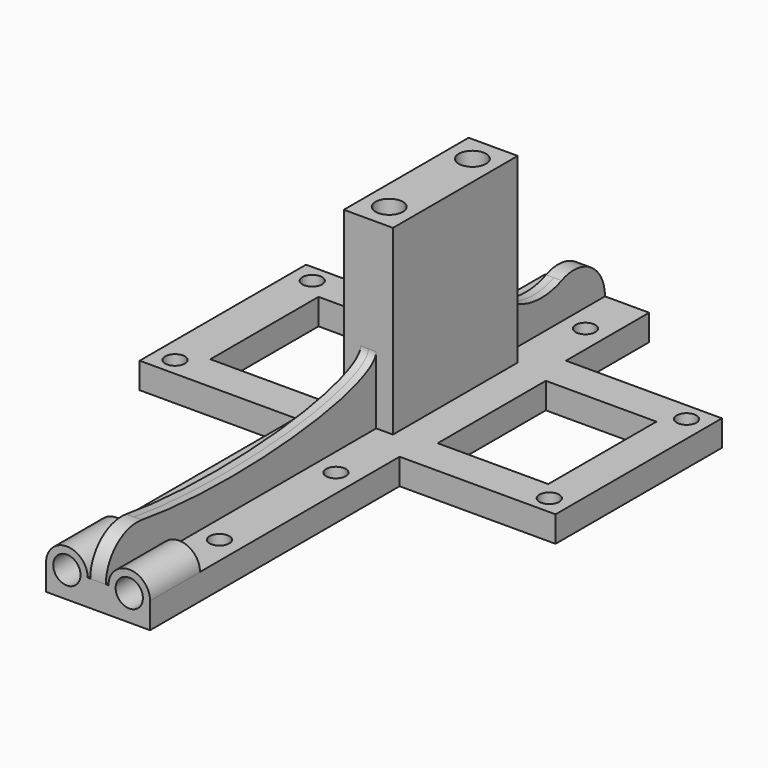
from build123d import *

# Parameters (mm, degrees)
F0_W      = 12
F0_H      = 38.1
F1_DEPTH  = 50.8
F2_R      = 3.33175
F3_DEPTH  = 25.4
F4_W      = 25.4
F4_H      = 76.2
F4_W_2    = 38.1
F4_H_2    = 50.8
F4_W_3    = 12
F4_H_3    = 38.1
F4_H_4    = 25.4
F5_DEPTH  = 6.35
F7_DEPTH  = 1.905
F8_R      = 3.33175
F9_DEPTH  = 12.7
F10_R     = 5.08
F11_DEPTH = 15.24
F13_DEPTH = 2.54
F14_W     = 27.02
F14_H     = 33.02
F15_DEPTH = 6.351
F16_R     = 2.413
F17_DEPTH = 6.351


# Not quite as in the source:
# - a pattern or mirror of a feature is missing from the dataset's text; its kind, count and spacing are read off the source's solid


with BuildPart() as f1:
    # F0 (on Top) → F1 (new body)
    with BuildSketch(Plane.XY):
        Rectangle(F0_W, F0_H)
    extrude(amount=F1_DEPTH)

    # F2 (on face) → F3 (cut)
    with BuildSketch(Plane.XY.offset(50.8)):
        with Locations((0, 12.7)):
            Circle(F2_R)
        with Locations((0, -12.7)):
            Circle(F2_R)
    extrude(amount=-F3_DEPTH, mode=Mode.SUBTRACT)

    # F4 (on face) → F5 (join)
    with BuildSketch(Plane(origin=(0, 0, 0), x_dir=(1, 0, 0), z_dir=(0, 0, -1))):
        with Locations((0, 63.5)):
            Rectangle(F4_W, F4_H)
        with Locations((31.75, 0)):
            Rectangle(F4_W_2, F4_H_2)
        Rectangle(F4_W, F4_H_2)
        Rectangle(F4_W_3, F4_H_3, mode=Mode.SUBTRACT)
        with Locations((-31.75, 0)):
            Rectangle(F4_W_2, F4_H_2)
        with Locations((0, -38.1)):
            Rectangle(F4_W, F4_H_4)
    extrude(amount=-F5_DEPTH)

    # F6 (on Right) → F7 (join, symmetric)
    with BuildSketch(Plane.YZ):
        with BuildLine():
            Line((-19.05, 6.35), (-19.05, 22.86))
            add(Edge.make_bspline(
                [(-90.6148681487, 15.7624194539), (-19.05, 4.6606890297), (-19.05, 22.86)],
                knots=[4.0563179373, 4.0563179373, 4.0563179373, 6.2831853072, 6.2831853072, 6.2831853072], degree=2, weights=[1, 0.4415833544, 1]))
            ThreePointArc((-90.6148681487, 15.7624194539), (-98.2724942161, 13.5830277507), (-101.6, 6.35))
            Line((-101.6, 6.35), (-25.4, 6.35))
            Line((-25.4, 6.35), (-19.05, 6.35))
        make_face()
        with BuildLine():
            Line((19.05, 22.86), (19.05, 6.35))
            Line((19.05, 6.35), (25.4, 6.35))
            Line((25.4, 6.35), (50.8, 6.35))
            ThreePointArc((50.8, 6.35), (46.5346393393, 14.2911472106), (37.5586731715, 15.1200934946))
            add(Edge.make_bspline(
                [(19.05, 22.86), (19.05, 7.2770438497), (37.5586731715, 15.1200934946)],
                knots=[0, 0, 0, 2.0982208016, 2.0982208016, 2.0982208016], degree=2, weights=[1, 0.4983425099, 1]))
        make_face()
    extrude(amount=F7_DEPTH, both=True)

    # F8 (on face) → F9 (cut)
    with BuildSketch(Plane.XZ.offset(101.6)):
        with Locations((-7.62, 6.35)):
            Circle(F8_R)
        with Locations((7.62, 6.35)):
            Circle(F8_R)
    extrude(amount=-F9_DEPTH, mode=Mode.SUBTRACT)

    # F10 (on face) → F11 (join)
    with BuildSketch(Plane.XZ.offset(101.6)):
        with Locations((-7.62, 6.35)):
            Circle(F10_R)
        with BuildLine():
            ThreePointArc((-4.28825, 6.35), (-7.62, 3.01825), (-10.95175, 6.35))
            ThreePointArc((-10.95175, 6.35), (-7.62, 9.68175), (-4.28825, 6.35))
        make_face(mode=Mode.SUBTRACT)
        with Locations((7.62, 6.35)):
            Circle(F10_R)
        with BuildLine():
            ThreePointArc((10.95175, 6.35), (7.62, 3.01825), (4.28825, 6.35))
            ThreePointArc((4.28825, 6.35), (7.62, 9.68175), (10.95175, 6.35))
        make_face(mode=Mode.SUBTRACT)
    extrude(amount=-F11_DEPTH)

    # F12 (on face) → F13 (join)
    with BuildSketch(Plane(origin=(0, -86.36, 0), x_dir=(-1, 0, 0), z_dir=(0, 1, 0))):
        with BuildLine():
            ThreePointArc((-4.28825, 6.35), (-7.62, 9.68175), (-10.95175, 6.35))
            Line((-10.95175, 6.35), (-4.28825, 6.35))
        make_face()
        with BuildLine():
            ThreePointArc((10.95175, 6.35), (7.62, 9.68175), (4.28825, 6.35))
            Line((4.28825, 6.35), (10.95175, 6.35))
        make_face()
    extrude(amount=-F13_DEPTH)

    # F14 (on face) → F15 (cut, through all)
    with BuildSketch(Plane.XY.offset(6.35)):
        with Locations((-27.13, 0)):
            Rectangle(F14_W, F14_H)
        with Locations((28.4, 0)):
            Rectangle(F14_W, F14_H)
    extrude(amount=-F15_DEPTH, mode=Mode.SUBTRACT)

    # F16 (on face) → F17 (cut, through all)
    with BuildSketch(Plane.XY.offset(6.35)):
        with Locations((-7.3025, -73.66)):
            Circle(F16_R)
        with Locations((-7.3025, -38.1)):
            Circle(F16_R)
        with Locations((-45.72, -20.955)):
            Circle(F16_R)
        with Locations((-45.72, 20.955)):
            Circle(F16_R)
        with Locations((-7.3025, 38.1)):
            Circle(F16_R)
    f17 = extrude(amount=-F17_DEPTH, mode=Mode.SUBTRACT)

    # F17_copies: F17 across plane
    add(f17.mirror(Plane(origin=(0, 0, 0), x_dir=(0, 0, 1), z_dir=(1, 0, 0))), mode=Mode.SUBTRACT)


solid = f1.part
